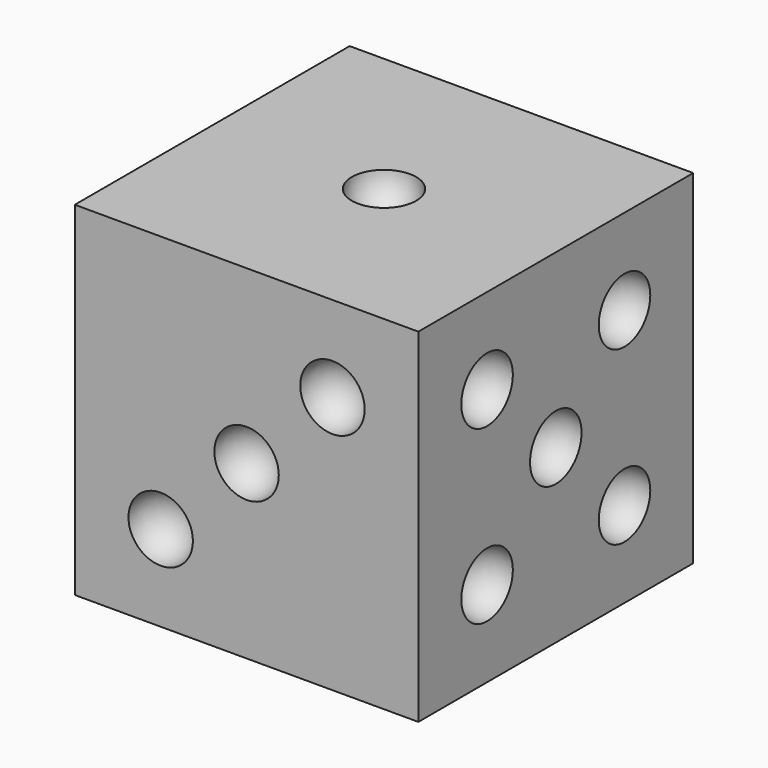
from build123d import *

# Parameters (mm, degrees)
F0_W      = 25.4
F0_H      = 25.4
F1_DEPTH  = 25.4
F2_R      = 2.38125
F3_DEPTH  = 2.38125
F4_R      = 2.38124
F5_R      = 2.38125
F6_DEPTH  = 2.38125
F7_R      = 2.38124
F8_R      = 2.38125
F9_DEPTH  = 2.38125
F10_R     = 2.38124
F11_R     = 2.38125
F12_DEPTH = 2.38125
F13_R     = 2.38124
F14_R     = 2.38125
F15_DEPTH = 2.38125
F16_R     = 2.38124
F17_R     = 2.38125
F18_DEPTH = 2.1166666667
F19_R     = 2.116657


# Not quite as in the source:
# - a fillet or chamfer is up to 0.001 mm smaller than in the source, because OpenCascade refuses the exact size


with BuildPart() as f1:
    # F0 (on Front) → F1 (new body)
    with BuildSketch(Plane.XZ):
        with Locations((12.7, 12.7)):
            Rectangle(F0_W, F0_H)
    extrude(amount=-F1_DEPTH)

    # F2 (on face) → F3 (cut)
    with BuildSketch(Plane.XZ):
        with Locations((6.35, 6.35)):
            Circle(F2_R)
        with Locations((12.7, 12.7)):
            Circle(F2_R)
        with Locations((19.05, 19.05)):
            Circle(F2_R)
    extrude(amount=-F3_DEPTH, mode=Mode.SUBTRACT)

    # F4 (radius 2.38125 in the source; OpenCascade refuses exactly that, so slightly less here)
    f4_edges = [f1.edges().sort_by_distance(p)[0] for p in [
        (16.66875, 2.38125, 19.05),
        (10.31875, 2.38125, 12.7),
        (3.96875, 2.38125, 6.35),
    ]]
    fillet(f4_edges, radius=F4_R)

    # F5 (on face) → F6 (cut)
    with BuildSketch(Plane.YZ.offset(25.4)):
        with Locations((12.7, 12.7)):
            Circle(F5_R)
        with Locations((6.35, 19.05)):
            Circle(F5_R)
        with Locations((6.35, 6.35)):
            Circle(F5_R)
        with Locations((19.05, 19.05)):
            Circle(F5_R)
        with Locations((19.05, 6.35)):
            Circle(F5_R)
    extrude(amount=-F6_DEPTH, mode=Mode.SUBTRACT)

    # F7 (radius 2.38125 in the source; OpenCascade refuses exactly that, so slightly less here)
    f7_edges = [f1.edges().sort_by_distance(p)[0] for p in [
        (23.01875, 3.96875, 19.05),
        (23.01875, 16.66875, 6.35),
        (23.01875, 16.66875, 19.05),
        (23.01875, 10.31875, 12.7),
        (23.01875, 3.96875, 6.35),
    ]]
    fillet(f7_edges, radius=F7_R)

    # F8 (on face) → F9 (cut)
    with BuildSketch(Plane.XY.offset(25.4)):
        with Locations((12.7, 12.7)):
            Circle(F8_R)
    extrude(amount=-F9_DEPTH, mode=Mode.SUBTRACT)

    # F10 (radius 2.38125 in the source; OpenCascade refuses exactly that, so slightly less here)
    f10_edges = [f1.edges().sort_by_distance(p)[0] for p in [
        (10.31875, 12.7, 23.01875),
    ]]
    fillet(f10_edges, radius=F10_R)

    # F11 (on face) → F12 (cut)
    with BuildSketch(Plane(origin=(0, 0, 0), x_dir=(1, 0, 0), z_dir=(0, 0, -1))):
        with Locations((6.35, -6.35)):
            Circle(F11_R)
        with Locations((6.35, -19.05)):
            Circle(F11_R)
        with Locations((19.05, -6.35)):
            Circle(F11_R)
        with Locations((19.05, -19.05)):
            Circle(F11_R)
    extrude(amount=-F12_DEPTH, mode=Mode.SUBTRACT)

    # F13 (radius 2.38125 in the source; OpenCascade refuses exactly that, so slightly less here)
    f13_edges = [f1.edges().sort_by_distance(p)[0] for p in [
        (3.96875, 6.35, 2.38125),
        (16.66875, 6.35, 2.38125),
        (16.66875, 19.05, 2.38125),
        (3.96875, 19.05, 2.38125),
    ]]
    fillet(f13_edges, radius=F13_R)

    # F14 (on face) → F15 (cut)
    with BuildSketch(Plane(origin=(0, 25.4, 0), x_dir=(-1, 0, 0), z_dir=(0, 1, 0))):
        with Locations((-19.05, 19.05)):
            Circle(F14_R)
        with Locations((-6.35, 6.35)):
            Circle(F14_R)
    extrude(amount=-F15_DEPTH, mode=Mode.SUBTRACT)

    # F16 (radius 2.38125 in the source; OpenCascade refuses exactly that, so slightly less here)
    f16_edges = [f1.edges().sort_by_distance(p)[0] for p in [
        (21.43125, 23.01875, 19.05),
        (8.73125, 23.01875, 6.35),
    ]]
    fillet(f16_edges, radius=F16_R)

    # F17 (on face) → F18 (cut)
    with BuildSketch(Plane(origin=(0, 0, 0), x_dir=(0, -1, 0), z_dir=(-1, 0, 0))):
        with Locations((-19.05, 19.05)):
            Circle(F17_R)
        with Locations((-19.05, 6.35)):
            Circle(F17_R)
        with Locations((-19.05, 12.7)):
            Circle(F17_R)
        with Locations((-6.35, 19.05)):
            Circle(F17_R)
        with Locations((-6.35, 12.7)):
            Circle(F17_R)
        with Locations((-6.35, 6.35)):
            Circle(F17_R)
    extrude(amount=-F18_DEPTH, mode=Mode.SUBTRACT)

    # F19 (radius 2.1166666667 in the source; OpenCascade refuses exactly that, so slightly less here)
    f19_edges = [f1.edges().sort_by_distance(p)[0] for p in [
        (2.116667, 21.43125, 19.05),
        (2.116667, 21.43125, 12.7),
        (2.116667, 21.43125, 6.35),
        (2.116667, 8.73125, 19.05),
        (2.116667, 8.73125, 12.7),
        (2.116667, 8.73125, 6.35),
    ]]
    fillet(f19_edges, radius=F19_R)


solid = f1.part
